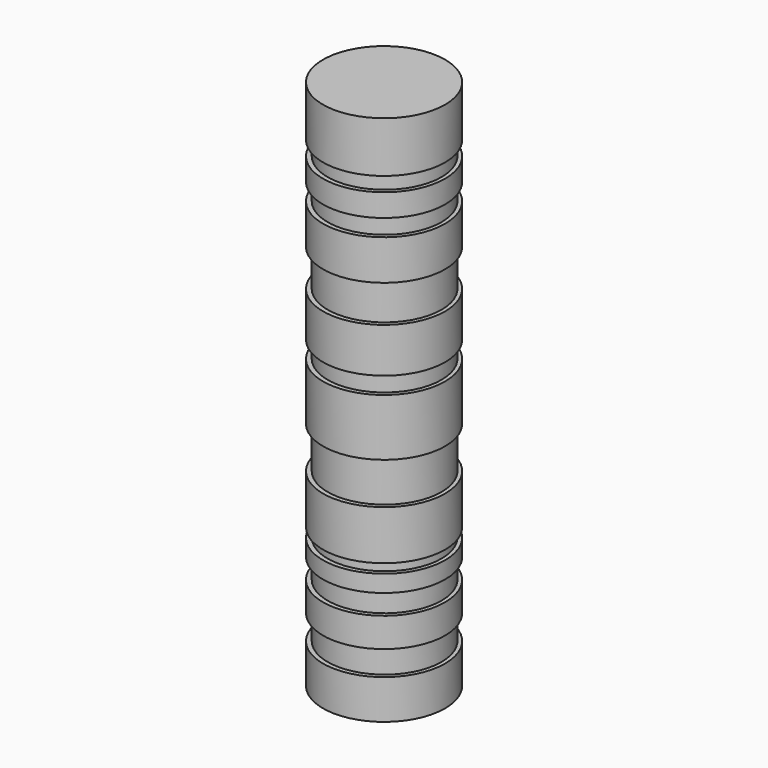
from build123d import *

# Parameters (mm, degrees)
F0_R     = 11.4835992145
F0_R_2   = 10.7107701276
F1_DEPTH = 100
F2_W     = 32.8816715628
F2_H     = 2.6963576674
F2_W_2   = 32.8778307885
F2_H_2   = 3.1931251287
F2_W_3   = 32.5816031545
F2_H_3   = 6.9668218493
F2_W_4   = 32.9470410943
F2_H_4   = 3.193128854
F2_W_5   = 29.896620661
F2_H_5   = 7.8376792371
F2_H_6   = 1.7417054623
F2_W_6   = 27.0034540445
F2_H_7   = 3.7736967206
F2_W_7   = 26.4959204942
F2_H_8   = 4.6445494518
F4_DEPTH = 100


# Not quite as in the source:
# - a feature names something its author has since deleted; it is built from what else it names


with BuildPart() as f1:
    # F0 (on Top) → F1 (new body)
    with BuildSketch(Plane.XY):
        with Locations((-0.0411355359, -0.0693021866)):
            Circle(F0_R)
        Circle(F0_R_2, mode=Mode.SUBTRACT)
    extrude(amount=F1_DEPTH)

    # F2 (on Front) → F3 (revolve, cut)
    with BuildSketch(Plane.XZ):
        with Locations((-16.4408357814, 89.0894643962)):
            Rectangle(F2_W, F2_H)
        with Locations((-16.4389153942, 81.8779617548)):
            Rectangle(F2_W_2, F2_H_2)
        with Locations((-16.2908015773, 69.2505948246)):
            Rectangle(F2_W_3, F2_H_3)
        with Locations((-16.4735205472, 55.7523723692)):
            Rectangle(F2_W_4, F2_H_4)
        with Locations((-14.9483103305, 39.4964460284)):
            Rectangle(F2_W_5, F2_H_5)
        with Locations((-14.9483103305, 25.4176529124)):
            Rectangle(F2_W_5, F2_H_6)
        with Locations((-13.5017270222, 19.4668248296)):
            Rectangle(F2_W_6, F2_H_7)
        with Locations((-13.2479602471, 9.7422976978)):
            Rectangle(F2_W_7, F2_H_8)
    revolve(axis=Axis((0, 0, 49.8652271926), (0, 0, 1)), mode=Mode.SUBTRACT)

    # F0 (on Top) → F4 (join)
    with BuildSketch(Plane.XY):
        Circle(F0_R_2)
    extrude(amount=F4_DEPTH)


solid = f1.part
